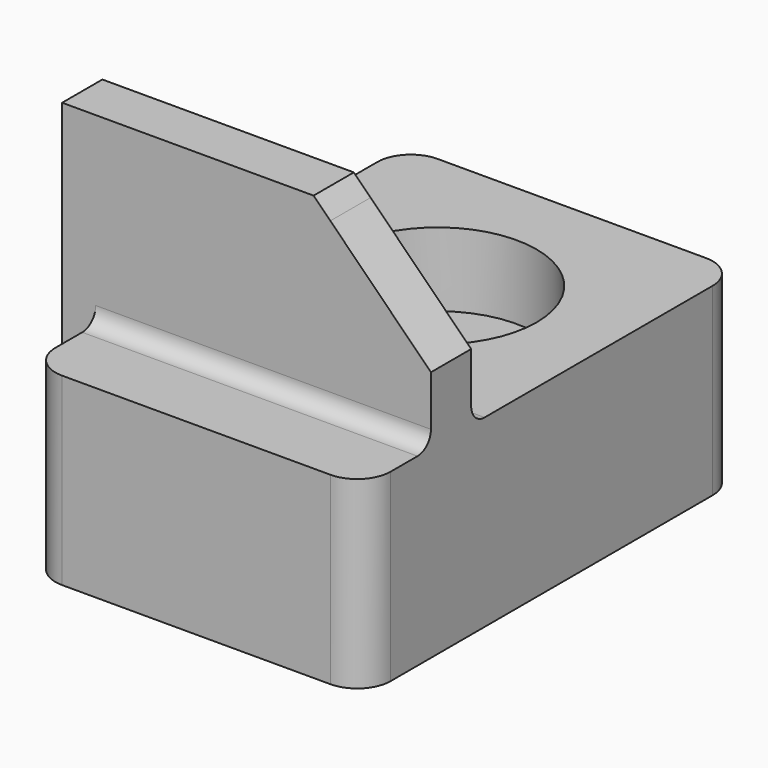
from build123d import *

# Parameters (mm, degrees)
F0_W           = 10
F0_H           = 14
F1_DEPTH       = 5.5
F4_D           = 2.83
F4_CBORE_D     = 5.9
F4_CBORE_DEPTH = 2.2
F2_W           = 8
F2_H           = 1.5
F5_DEPTH       = 11
F6_SIZE        = 1
F7_R           = 1
F8_T4_DEPTH    = 1.5
F9_SIZE        = 0.49999
F10_R          = 0.5


# Not quite as in the source:
# - a fillet or chamfer that OpenCascade refuses, or shapes differently, is made with other operations: its cross-section is extruded or revolved along the edge and cut away or added
# - a fillet or chamfer is up to 0.001 mm smaller than in the source, because OpenCascade refuses the exact size


with BuildPart() as f1:
    # F0 (on Top) → F1 (new body)
    with BuildSketch(Plane.XY):
        with Locations((5, 7)):
            Rectangle(F0_W, F0_H)
    extrude(amount=F1_DEPTH)

    # F4 (through all)
    with Locations(Plane.XY.offset(5.5)):
        with Locations((5, 9)):
            CounterBoreHole(F4_D / 2, F4_CBORE_D / 2, F4_CBORE_DEPTH)

    # F2 (on Top) → F5 (join)
    with BuildSketch(Plane.XY):
        with Locations((3, 3.25)):
            Rectangle(F2_W, F2_H)
    extrude(amount=F5_DEPTH)

    # F6
    f6_edges = [f1.edges().sort_by_distance(p)[0] for p in [
        (-1, 3.25, 0),
    ]]
    chamfer(f6_edges, length=F6_SIZE)

    # F7
    f7_edges = [f1.edges().sort_by_distance(p)[0] for p in [
        (0, 14, 2.75),
        (10, 14, 2.75),
        (10, 0, 2.75),
        (0, 0, 2.75),
    ]]
    fillet(f7_edges, radius=F7_R)

    # F8: chamfer of 5 on 1 edges, made by hand


with BuildPart() as f8_tool2:
    # F8_s3 → F8_t4 (new body)
    with BuildSketch(Plane.XZ.offset(-4)):
        Polygon((12, 5.5), (7, 10.5), (7, 5.5), align=None)
    extrude(amount=F8_T4_DEPTH)

    split(bisect_by=Plane.YZ.offset(10), keep=Keep.BOTTOM)


with BuildPart() as f1_1:
    add(f1.part)

    # F8_t1: union F8_tool2
    add(f8_tool2.part)

    # F9 (size 0.5 in the source; OpenCascade refuses exactly that, so slightly less here)
    f9_edges = [f1_1.edges().sort_by_distance(p)[0] for p in [
        (7, 3.25, 11),
    ]]
    chamfer(f9_edges, length=F9_SIZE)

    # F10
    f10_edges = [f1_1.edges().sort_by_distance(p)[0] for p in [
        (5, 4, 5.5),
        (5, 2.5, 5.5),
    ]]
    fillet(f10_edges, radius=F10_R)


solid = f1_1.part
